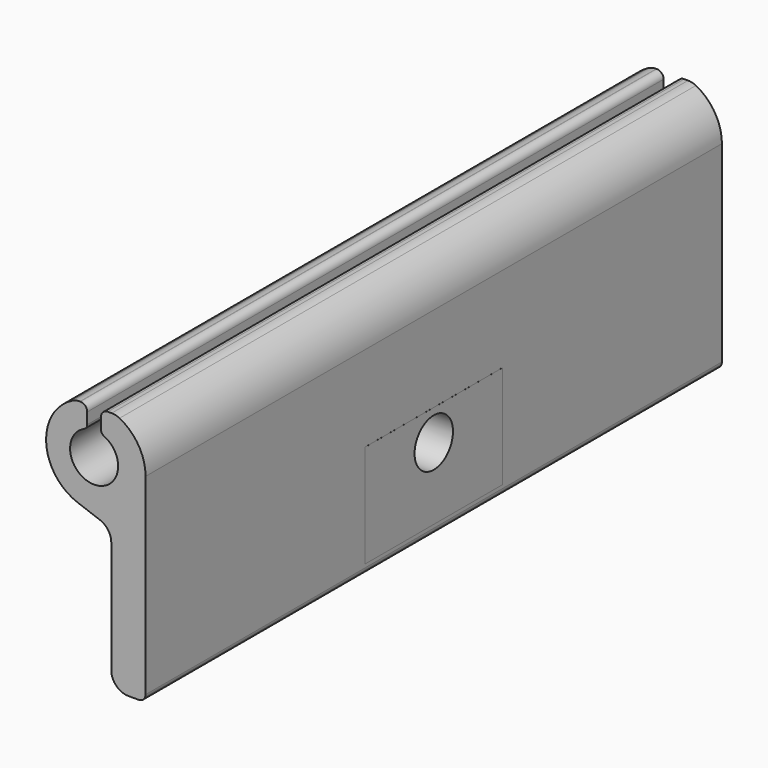
from build123d import *

# Parameters (mm, degrees)
F1_DEPTH = 105
F2_R     = 12
F2_R_2   = 7
F3_DEPTH = 0.01
F4_W     = 50
F4_H     = 30
F5_DEPTH = 0.01
F6_DEPTH = 20


# Not quite as in the source:
# - ends of sketch curves that miss each other by under 0.0002 mm in the source are joined


with BuildPart() as f1:
    # F0 (on Front) → F1 (new body, symmetric)
    with BuildSketch(Plane.XZ):
        with BuildLine():
            Line((4.4999999997, -23.5), (4.4999999997, -30.5))
            ThreePointArc((4.4999999997, -30.5), (5.9644660938, -34.0355339059), (9.4999999997, -35.5))
            Line((9.4999999997, -35.5), (12.5, -35.5))
            ThreePointArc((12.5, -35.5), (13.9142133287, -34.9142135624), (14.4999997663, -33.5))
            Line((14.4999997663, -33.5), (14.4999997663, 22.4999994828))
            ThreePointArc((14.4999997663, 22.4999994828), (12.4539129776, 29.7872458033), (6.9137199183, 34.9444437777))
            ThreePointArc((6.9137199183, 34.9444437777), (5.8016169865, 35.3591259101), (4.6231056877, 35.4999993303))
            Line((4.6231056877, 35.4999993303), (3.4999997663, 35.4999993303))
            ThreePointArc((3.4999997663, 35.4999993303), (2.0857862039, 34.9142128927), (1.4999997663, 33.4999993303))
            Line((1.4999997663, 33.4999993303), (1.4999997663, 30.2459664828))
            ThreePointArc((1.4999997663, 30.2459664828), (1.7397477835, 29.4324771221), (2.3823530195, 28.8790310431))
            ThreePointArc((2.3823530195, 28.8790310431), (-0.5000000985, 15.4999997293), (-3.3823532363, 28.8790310342))
            ThreePointArc((-3.3823532363, 28.8790310342), (-2.7397478169, 29.4324771961), (-2.4999997997, 30.2459665567))
            Line((-2.4999997997, 30.2459665567), (-2.4999997997, 33.5))
            ThreePointArc((-2.4999997997, 33.5), (-3.0857862373, 34.9142132361), (-4.4999997997, 35.4999996738))
            Line((-4.4999997997, 35.4999996738), (-4.6231058319, 35.4999996738))
            ThreePointArc((-4.6231058319, 35.4999996738), (-5.8016171306, 35.3591262536), (-6.9137200625, 34.9444441212))
            ThreePointArc((-6.9137200625, 34.9444441212), (-14.4718653147, 21.6128794539), (-5.288282, 9.344303))
            Line((-5.288282, 9.344303), (1.210101, 6.979085))
            ThreePointArc((1.210101, 6.979085), (3.5957603078, 5.1485040574), (4.4999999997, 2.2806219993))
            Line((4.4999999997, 2.2806219993), (4.4999999997, 0.5))
            Line((4.4999999997, 0.5), (4.4999999997, -23.5))
        make_face()
    extrude(amount=F1_DEPTH, both=True)

    # F2 (on face) → F3 (join)
    with BuildSketch(Plane(origin=(4.4999999997, 0, 0), x_dir=(0, -1, 0), z_dir=(-1, 0, 0))):
        with Locations((0, -11.5)):
            Circle(F2_R)
        with Locations((0, -11.5)):
            Circle(F2_R_2, mode=Mode.SUBTRACT)
    extrude(amount=F3_DEPTH)

    # F4 (on face) → F5 (join)
    with BuildSketch(Plane.YZ.offset(14.4999997663)):
        with Locations((0, -17.5000005172)):
            Rectangle(F4_W, F4_H)
    extrude(amount=F5_DEPTH)

    # F6 (cut): a face of the model
    f6_faces = [f1.faces().sort_by_distance(p)[0] for p in [
        (4.4999999997, 0, -11.5),
    ]]
    extrude(f6_faces, amount=-F6_DEPTH, mode=Mode.SUBTRACT)


solid = f1.part
